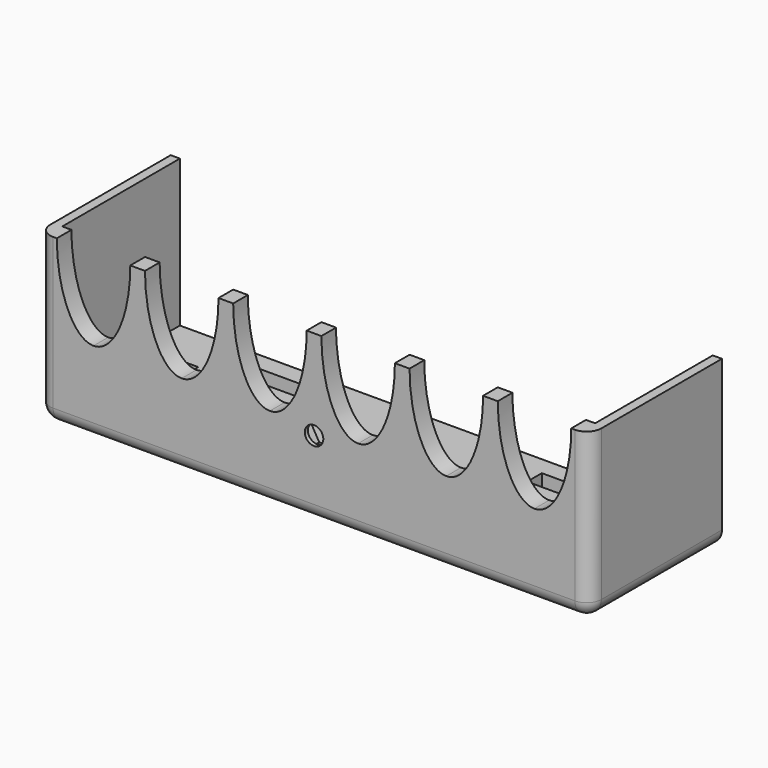
from build123d import *

# Parameters (mm, degrees)
F0_W          = 190.5
F0_H          = 57.15
F0_W_2        = 31.75
F0_H_2        = 6.35
F1_DEPTH      = 6.35
F3_DEPTH      = 50.8
F4_R          = 1.575
F5_DEPTH      = 25.4
F6_R          = 3
F7_DEPTH      = 3.25
F9_DEPTH      = 5
F10_R         = 3.2
F11_DEPTH     = 25.4
F12_W         = 19.05
F12_H         = 25.4
F13_DEPTH     = 25.4
F14_T1_DEPTH  = 64.77
F14_T3_DEPTH  = 64.77
F14_T5_DEPTH  = 180.34
F14_S9_W      = 5.08
F14_S9_H      = 5.08
F14_T10_DEPTH = 5.08
F14_S15_W     = 5.08
F14_S15_H     = 5.08
F14_T16_DEPTH = 5.08
F16_DEPTH     = 6.351


# Not quite as in the source:
# - a fillet or chamfer that OpenCascade refuses, or shapes differently, is made with other operations: its cross-section is extruded or revolved along the edge and cut away or added


with BuildPart() as f1:
    # F0 (on Top) → F1 (new body)
    with BuildSketch(Plane.XY):
        with Locations((0, -49.0298296415)):
            Rectangle(F0_W, F0_H)
        with Locations((-53.975, -68.0798296415)):
            Rectangle(F0_W_2, F0_H_2, mode=Mode.SUBTRACT)
        with Locations((53.975, -68.0798296415)):
            Rectangle(F0_W_2, F0_H_2, mode=Mode.SUBTRACT)
        with Locations((-53.975, -29.9798296415)):
            Rectangle(F0_W_2, F0_H_2, mode=Mode.SUBTRACT)
        with Locations((53.975, -29.9798296415)):
            Rectangle(F0_W_2, F0_H_2, mode=Mode.SUBTRACT)
    extrude(amount=F1_DEPTH)

    # F2 (on face) → F3 (join)
    with BuildSketch(Plane.XY.offset(6.35)):
        Polygon((-92.075, -20.4548296415), (-95.25, -20.4548296415), (-95.25, -77.6048296415), (95.25, -77.6048296415), (95.25, -20.4548296415), (92.075, -20.4548296415), (92.075, -71.2548296415), (-92.075, -71.2548296415), align=None)
    extrude(amount=F3_DEPTH)

    # F4 (on face) → F5 (cut)
    with BuildSketch(Plane.XY.offset(6.35)):
        with Locations((-50, -53.2548296415)):
            Circle(F4_R)
        with Locations((50, -53.2548296415)):
            Circle(F4_R)
    extrude(amount=-F5_DEPTH, mode=Mode.SUBTRACT)

    # F6 (on face) → F7 (cut)
    with BuildSketch(Plane(origin=(0, 0, 0), x_dir=(1, 0, 0), z_dir=(0, 0, -1))):
        with Locations((-50, 53.2548296415)):
            Circle(F6_R)
        with Locations((50, 53.2548296415)):
            Circle(F6_R)
    extrude(amount=-F7_DEPTH, mode=Mode.SUBTRACT)

    # F8 (on face) → F9 (cut)
    with BuildSketch(Plane(origin=(0, -71.2548296415, 0), x_dir=(-1, 0, 0), z_dir=(0, 1, 0))):
        Polygon((3.2908965344, 20.35), (6.5817930688, 26.05), (3.2908965344, 31.75), (-3.2908965344, 31.75), (-6.5817930688, 26.05), (-3.2908965344, 20.35), align=None)
    extrude(amount=-F9_DEPTH, mode=Mode.SUBTRACT)

    # F10 (on face) → F11 (cut)
    with BuildSketch(Plane(origin=(0, -76.2548296415, 0), x_dir=(-1, 0, 0), z_dir=(0, 1, 0))):
        with Locations((0, 26.05)):
            Circle(F10_R)
    extrude(amount=-F11_DEPTH, mode=Mode.SUBTRACT)

    # F12 (on face) → F13 (cut)
    with BuildSketch(Plane(origin=(0, 0, 0), x_dir=(1, 0, 0), z_dir=(0, 0, -1))):
        with Locations((-82.55, 49.0298296415)):
            Rectangle(F12_W, F12_H)
        with Locations((82.55, 49.0298296415)):
            Rectangle(F12_W, F12_H)
    extrude(amount=-F13_DEPTH, mode=Mode.SUBTRACT)

    # F14: fillet of radius 5.08 on 5 edges, made by hand

    # F14_s2 → F14_t1 (cut)
    with BuildSketch(Plane.XZ.offset(7.7548296415)):
        with BuildLine():
            ThreePointArc((-90.17, 0), (-93.7621024484, 1.4878975516), (-95.25, 5.08))
            Line((-95.25, 5.08), (-95.25, 0))
            Line((-95.25, 0), (-90.17, 0))
        make_face()
        with BuildLine():
            ThreePointArc((95.25, 5.08), (93.7621024484, 1.4878975516), (90.17, 0))
            Line((90.17, 0), (95.25, 0))
            Line((95.25, 0), (95.25, 5.08))
        make_face()
    extrude(amount=F14_T1_DEPTH, mode=Mode.SUBTRACT)

    # F14_s4 → F14_t3 (cut)
    with BuildSketch(Plane.XY.offset(5.08)):
        with BuildLine():
            ThreePointArc((-90.17, -77.6048296415), (-93.7621024484, -76.1169320899), (-95.25, -72.5248296415))
            Line((-95.25, -72.5248296415), (-95.25, -77.6048296415))
            Line((-95.25, -77.6048296415), (-90.17, -77.6048296415))
        make_face()
        with BuildLine():
            ThreePointArc((95.25, -72.5248296415), (93.7621024484, -76.1169320899), (90.17, -77.6048296415))
            Line((90.17, -77.6048296415), (95.25, -77.6048296415))
            Line((95.25, -77.6048296415), (95.25, -72.5248296415))
        make_face()
    extrude(amount=F14_T3_DEPTH, mode=Mode.SUBTRACT)

    # F14_s6 → F14_t5 (cut)
    with BuildSketch(Plane.YZ.offset(-90.17)):
        with BuildLine():
            ThreePointArc((-77.6048296415, 5.08), (-76.1169320899, 1.4878975516), (-72.5248296415, 0))
            Line((-72.5248296415, 0), (-77.6048296415, 0))
            Line((-77.6048296415, 0), (-77.6048296415, 5.08))
        make_face()
    extrude(amount=F14_T5_DEPTH, mode=Mode.SUBTRACT)


with BuildPart() as f14_tool8:
    # F14_s9 → F14_t10 (new body)
    with BuildSketch(Plane.XZ.offset(72.5248296415)):
        with Locations((-92.71, 2.54)):
            Rectangle(F14_S9_W, F14_S9_H)
    extrude(amount=F14_T10_DEPTH)

    # F14_s11 → F14_t12 (revolve, cut)
    with BuildSketch(Plane(origin=(-90.17, -72.5248296415, 5.08), x_dir=(0.7071067812, 0, 0.7071067812), z_dir=(0.7071067812, 0, -0.7071067812))):
        with BuildLine():
            ThreePointArc((0, -5.08), (5.08, 0), (0, 5.08))
            Line((0, 5.08), (0, -5.08))
        make_face()
    revolve(axis=Axis((-90.17, -72.5248296415, 5.08), (0, -1, 0)), mode=Mode.SUBTRACT)


with BuildPart() as f1_1:
    add(f1.part)

    # F14_t7: cut F14_tool8
    add(f14_tool8.part, mode=Mode.SUBTRACT)


with BuildPart() as f14_tool14:
    # F14_s15 → F14_t16 (new body)
    with BuildSketch(Plane.YZ.offset(90.17)):
        with Locations((-75.0648296415, 2.54)):
            Rectangle(F14_S15_W, F14_S15_H)
    extrude(amount=F14_T16_DEPTH)

    # F14_s17 → F14_t18 (revolve, cut)
    with BuildSketch(Plane(origin=(90.17, -72.5248296415, 5.08), x_dir=(0, 0.7071067812, 0.7071067812), z_dir=(0, 0.7071067812, -0.7071067812))):
        with BuildLine():
            ThreePointArc((0, -5.08), (5.08, 0), (0, 5.08))
            Line((0, 5.08), (0, -5.08))
        make_face()
    revolve(axis=Axis((90.17, -72.5248296415, 5.08), (1, 0, 0)), mode=Mode.SUBTRACT)


with BuildPart() as f1_2:
    add(f1_1.part)

    # F14_t13: cut F14_tool14
    add(f14_tool14.part, mode=Mode.SUBTRACT)

    # F15 (on face) → F16 (cut, through all)
    with BuildSketch(Plane(origin=(0, -71.2548296415, 0), x_dir=(-1, 0, 0), z_dir=(0, 1, 0))):
        with BuildLine():
            add(Edge.make_bspline(
                [(-76.2, 28.575), (-54.2029547439, 28.575), (-65.2014773719, 71.4375), (-76.2, 114.3), (-87.1985226281, 71.4375), (-98.1970452561, 28.575), (-76.2, 28.575)],
                knots=[0, 0, 0, 2.0943951024, 2.0943951024, 4.1887902048, 4.1887902048, 6.2831853072, 6.2831853072, 6.2831853072], degree=2, weights=[1, 0.5, 1, 0.5, 1, 0.5, 1]))
        make_face()
        with BuildLine():
            add(Edge.make_bspline(
                [(-45.72, 28.575), (-23.7229547439, 28.575), (-34.7214773719, 71.4375), (-45.72, 114.3), (-56.7185226281, 71.4375), (-67.7170452561, 28.575), (-45.72, 28.575)],
                knots=[0, 0, 0, 2.0943951024, 2.0943951024, 4.1887902048, 4.1887902048, 6.2831853072, 6.2831853072, 6.2831853072], degree=2, weights=[1, 0.5, 1, 0.5, 1, 0.5, 1]))
        make_face()
        with BuildLine():
            add(Edge.make_bspline(
                [(-15.24, 28.575), (6.7570452561, 28.575), (-4.2414773719, 71.4375), (-15.24, 114.3), (-26.2385226281, 71.4375), (-37.2370452561, 28.575), (-15.24, 28.575)],
                knots=[0, 0, 0, 2.0943951024, 2.0943951024, 4.1887902048, 4.1887902048, 6.2831853072, 6.2831853072, 6.2831853072], degree=2, weights=[1, 0.5, 1, 0.5, 1, 0.5, 1]))
        make_face()
        with BuildLine():
            add(Edge.make_bspline(
                [(15.24, 28.575), (37.2370452561, 28.575), (26.2385226281, 71.4375), (15.24, 114.3), (4.2414773719, 71.4375), (-6.7570452561, 28.575), (15.24, 28.575)],
                knots=[0, 0, 0, 2.0943951024, 2.0943951024, 4.1887902048, 4.1887902048, 6.2831853072, 6.2831853072, 6.2831853072], degree=2, weights=[1, 0.5, 1, 0.5, 1, 0.5, 1]))
        make_face()
        with BuildLine():
            add(Edge.make_bspline(
                [(45.72, 28.575), (67.7170452561, 28.575), (56.7185226281, 71.4375), (45.72, 114.3), (34.7214773719, 71.4375), (23.7229547439, 28.575), (45.72, 28.575)],
                knots=[0, 0, 0, 2.0943951024, 2.0943951024, 4.1887902048, 4.1887902048, 6.2831853072, 6.2831853072, 6.2831853072], degree=2, weights=[1, 0.5, 1, 0.5, 1, 0.5, 1]))
        make_face()
        with BuildLine():
            add(Edge.make_bspline(
                [(76.2, 28.575), (98.1970452561, 28.575), (87.1985226281, 71.4375), (76.2, 114.3), (65.2014773719, 71.4375), (54.2029547439, 28.575), (76.2, 28.575)],
                knots=[0, 0, 0, 2.0943951024, 2.0943951024, 4.1887902048, 4.1887902048, 6.2831853072, 6.2831853072, 6.2831853072], degree=2, weights=[1, 0.5, 1, 0.5, 1, 0.5, 1]))
        make_face()
    extrude(amount=-F16_DEPTH, mode=Mode.SUBTRACT)


solid = f1_2.part
